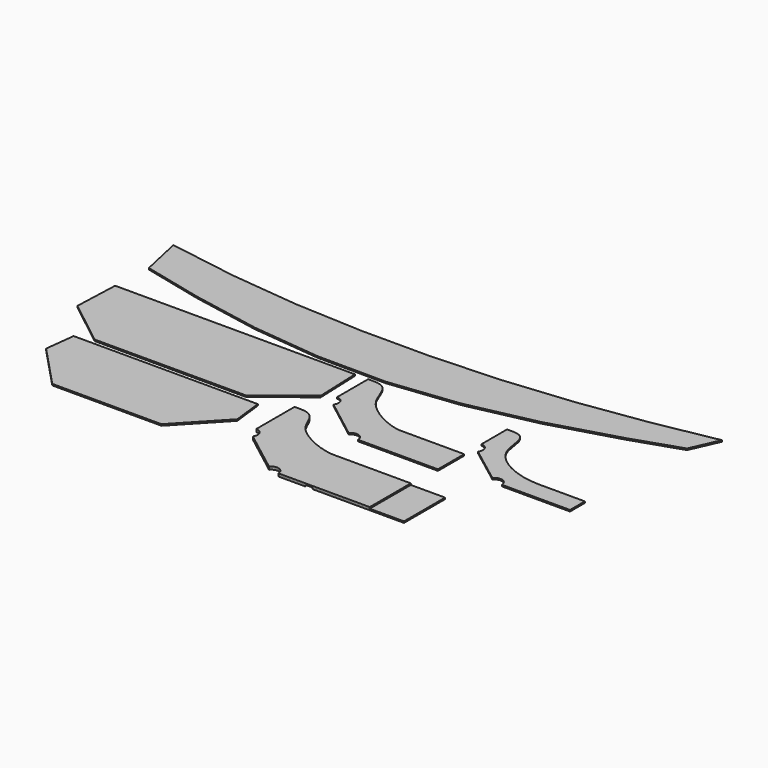
from build123d import *

# Parameters (mm, degrees)
F1_DEPTH = 6.35
F2_DEPTH = 6.35
F0_W     = 152.4
F0_H     = 228.6
F5_DEPTH = 6.35


with BuildPart() as f1:
    # F0 (on Top) → F1 (new body)
    with BuildSketch(Plane.XY):
        with BuildLine():
            Line((1184.275, -409.575), (1158.875, -409.575))
            Line((1158.875, -409.575), (1158.875, -582.6125))
            ThreePointArc((1158.875, -582.6125), (1187.3519406863, -600.3223308717), (1184.0605788026, -633.6950921795))
            Line((1184.0605788026, -633.6950921795), (1359.1144211974, -768.0674078205))
            ThreePointArc((1359.1144211974, -768.0674078205), (1394.5083390671, -757.3358633337), (1416.05, -787.4))
            Line((1416.05, -787.4), (1771.65, -787.4))
            Line((1771.65, -787.4), (1771.65, -641.35))
            Line((1771.65, -641.35), (1489.075, -641.35))
            add(Edge.make_bspline(
                [(1184.275, -409.575), (1260.475, -409.575), (1239.6705562427, -549.8166383278), (1438.275, -641.35), (1489.075, -641.35)],
                knots=[0, 0, 0, 0, 0.4480292942, 1, 1, 1, 1], degree=3))
        make_face()
    extrude(amount=F1_DEPTH)


with BuildPart() as f1b:
    # F0 (on Top) → F1, piece 2 (new body)
    with BuildSketch(Plane.XY):
        with BuildLine():
            Line((1517.65, -1166.8125), (1771.65, -1166.8125))
            Line((1771.65, -1166.8125), (1771.65, -938.2125))
            Line((1771.65, -938.2125), (1427.1625, -938.2125))
            add(Edge.make_bspline(
                [(1122.3625, -741.3625), (1198.5625, -741.3625), (1179.69287535, -863.0083351522), (1376.3625, -938.2125), (1427.1625, -938.2125)],
                knots=[0, 0, 0, 0, 0.441817609, 1, 1, 1, 1], degree=3))
            Line((1122.3625, -741.3625), (1096.9625, -741.3625))
            Line((1096.9625, -741.3625), (1096.9625, -954.0875))
            ThreePointArc((1096.9625, -954.0875), (1123.7331565008, -968.7672202566), (1125.7488052209, -999.231944062))
            Line((1125.7488052209, -999.231944062), (1457.1136947791, -1153.418055938))
            ThreePointArc((1457.1136947791, -1153.418055938), (1492.7592021853, -1135.8122766882), (1517.65, -1166.8125))
        make_face()
    extrude(amount=F1_DEPTH)


with BuildPart() as f1c:
    # F0 (on Top) → F1, piece 3 (new body)
    with BuildSketch(Plane.XY):
        with BuildLine():
            Line((1797.05, -403.0552663527), (1771.65, -403.0552663527))
            Line((1771.65, -403.0552663527), (1771.65, -545.9302663527))
            ThreePointArc((1771.65, -545.9302663527), (1800.0731941464, -563.5316079528), (1796.9822875345, -596.8202169344))
            Line((1796.9822875345, -596.8202169344), (1960.6302124655, -720.4653157711))
            ThreePointArc((1960.6302124655, -720.4653157711), (1996.0561210247, -709.5024207296), (2017.7125, -739.6052663527))
            Line((2017.7125, -739.6052663527), (2320.925, -739.6052663527))
            Line((2320.925, -739.6052663527), (2320.925, -657.0552663527))
            Line((2320.925, -657.0552663527), (2117.725, -657.0552663527))
            add(Edge.make_bspline(
                [(2117.725, -657.0552663527), (2016.125, -657.0552663527), (1820.8710671265, -570.1012868563), (1873.25, -403.0552663527), (1797.05, -403.0552663527)],
                knots=[0, 0, 0, 0, 0.5769629955, 1, 1, 1, 1], degree=3))
        make_face()
    extrude(amount=F1_DEPTH)


with BuildPart() as f1d:
    # F0 (on Top) → F1, piece 4 (new body)
    with BuildSketch(Plane.XY):
        Polygon((976.3125, -795.3375), (566.7375, -795.3375), (157.1625, -795.3375), (141.2875, -928.6875), (323.85, -1122.3625), (566.7375, -1122.3625), (809.625, -1122.3625), (992.1875, -928.6875), align=None)
    extrude(amount=F1_DEPTH)


with BuildPart() as f1e:
    # F0 (on Top) → F1, piece 5 (new body)
    with BuildSketch(Plane.XY):
        Polygon((566.7375, -409.575), (33.3375, -409.575), (25.4, -609.6), (230.1875, -769.9375), (566.7375, -769.9375), (903.2875, -769.9375), (1108.075, -609.6), (1100.1375, -409.575), align=None)
    extrude(amount=F1_DEPTH)


with BuildPart() as f1f:
    # F0 (on Top) → F1, piece 6 (new body)
    with BuildSketch(Plane.XY):
        Polygon((304.8, -93.6625), (0, -44.45), (41.275, -232.1388020833), (304.8, -295.275), (609.6, -352.425), (914.4, -384.175), (1219.2, -385.7625), (1524, -350.8375), (1828.8, -285.75), (2133.6, -196.85), (2349.5, -124.8833333333), (2405.0625, 0), (2133.6, -50.8), (1828.8, -95.25), (1524, -125.4125), (1219.2, -139.7), (914.4, -139.7), (609.6, -125.4125), align=None)
    extrude(amount=F1_DEPTH)


with BuildPart() as f2:
    # F0 (on Top) → F2 (new body)
    with BuildSketch(Plane.XY):
        with BuildLine():
            Line((1365.25, -1166.8125), (1485.9, -1166.8125))
            Line((1485.9, -1166.8125), (1457.1136947791, -1153.418055938))
            Line((1457.1136947791, -1153.418055938), (1125.7488052209, -999.231944062))
            ThreePointArc((1125.7488052209, -999.231944062), (1124.124265246, -1002.2783335774), (1122.1785567933, -1005.130321976))
            Line((1122.1785567933, -1005.130321976), (1308.2839432067, -1147.519678024))
            ThreePointArc((1308.2839432067, -1147.519678024), (1343.6846133165, -1136.740317645), (1365.25, -1166.8125))
        make_face()
    extrude(amount=F2_DEPTH)


with BuildPart() as f2b:
    # F0 (on Top) → F2, piece 2 (new body)
    with BuildSketch(Plane.XY):
        with Locations((1847.85, -1052.5125)):
            Rectangle(F0_W, F0_H)
    extrude(amount=F2_DEPTH)


with BuildPart() as f5:
    # F4 (on face) → F5 (new body)
    with BuildSketch(Plane.XY.offset(6.35)):
        with BuildLine():
            Line((1096.9625, -741.3625), (1096.9625, -954.0875))
            ThreePointArc((1096.9625, -954.0875), (1102.5763225769, -954.5877400637), (1108.0132469514, -956.0726970977))
            Line((1108.0132469514, -956.0726970977), (1675.633582901, -1166.8125))
            Line((1675.633582901, -1166.8125), (1771.65, -1166.8125))
            Line((1771.65, -1166.8125), (1771.65, -938.2125))
            Line((1771.65, -938.2125), (1427.1625, -938.2125))
            add(Edge.make_bspline(
                [(1195.3044928639, -785.2942482262), (1188.3905985456, -810.7493696117), (1146.6295208593, -926.9508572649), (1326.0216633776, -937.4958061878), (1411.7701730659, -939.0812615273), (1427.1625, -938.2125)],
                knots=[127.292389292, 127.292389292, 127.292389292, 127.292389292, 199.3006577737, 409.8585065241, 460.6585065241, 460.6585065241, 460.6585065241, 460.6585065241], degree=3))
            add(Edge.make_bspline(
                [(1122.3625, -741.3625), (1167.7508107351, -741.3625), (1183.1457987153, -760.4310803701), (1195.3044928639, -785.2942482262)],
                knots=[0, 0, 0, 0, 0.2631673875, 0.2631673875, 0.2631673875, 0.2631673875], degree=3))
            Line((1122.3625, -741.3625), (1096.9625, -741.3625))
        make_face()
        with BuildLine():
            Line((1675.633582901, -1166.8125), (1108.0132469514, -956.0726970977))
            ThreePointArc((1108.0132469514, -956.0726970977), (1126.3296216001, -973.7695810028), (1125.7488052209, -999.231944062))
            ThreePointArc((1125.7488052209, -999.231944062), (1124.124265246, -1002.2783335774), (1122.1785567933, -1005.130321976))
            Line((1122.1785567933, -1005.130321976), (1308.2839432067, -1147.519678024))
            ThreePointArc((1308.2839432067, -1147.519678024), (1343.6846133165, -1136.740317645), (1365.25, -1166.8125))
            Line((1365.25, -1166.8125), (1485.9, -1166.8125))
            Line((1485.9, -1166.8125), (1517.65, -1166.8125))
            Line((1517.65, -1166.8125), (1675.633582901, -1166.8125))
        make_face()
        with BuildLine():
            add(Edge.make_bspline(
                [(1195.3044928639, -785.2942482262), (1203.5583780583, -802.1725190786), (1231.4499066642, -882.7996187422), (1376.3625, -938.2125), (1427.1625, -938.2125)],
                knots=[0.2631673875, 0.2631673875, 0.2631673875, 0.2631673875, 0.441817609, 1, 1, 1, 1], degree=3))
            add(Edge.make_bspline(
                [(1195.3044928639, -785.2942482262), (1188.3905985456, -810.7493696117), (1146.6295208593, -926.9508572649), (1326.0216633776, -937.4958061878), (1411.7701730659, -939.0812615273), (1427.1625, -938.2125)],
                knots=[127.292389292, 127.292389292, 127.292389292, 127.292389292, 199.3006577737, 409.8585065241, 460.6585065241, 460.6585065241, 460.6585065241, 460.6585065241], degree=3))
        make_face()
    extrude(amount=F5_DEPTH)


solid = Compound([f1.part, f1b.part, f1c.part, f1d.part, f1e.part, f1f.part, f2.part, f2b.part, f5.part])
